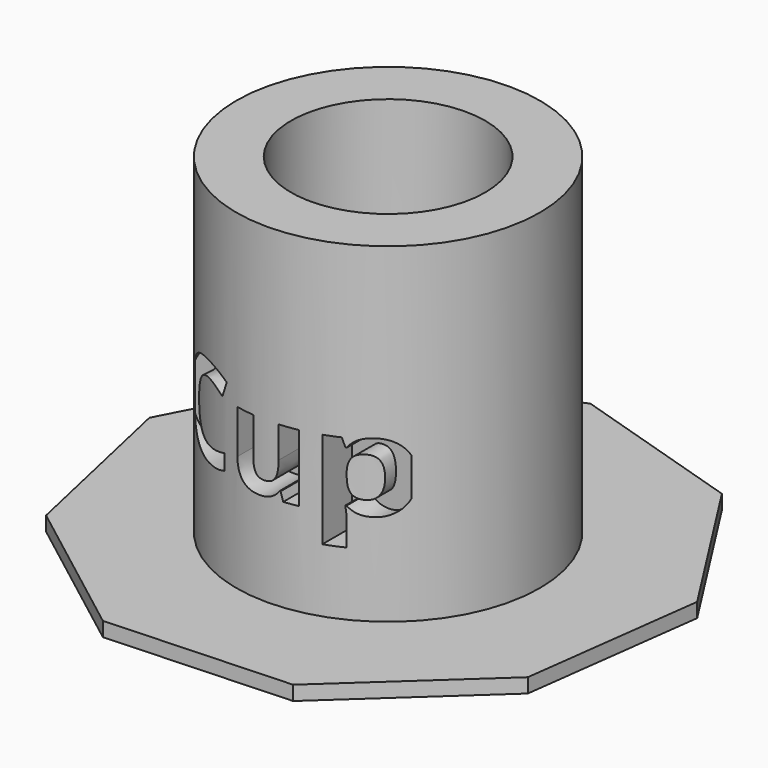
from build123d import *

# Parameters (mm, degrees)
F0_R         = 67.0452350449
F1_DEPTH     = 152.4
F2_T         = -24.13
F4_TEXT_SIZE = 54.2367187639
F5_DEPTH     = 21.59
F7_DEPTH     = 6.35


# Not quite as in the source:
# - a feature names something its author has since deleted; it is built from what else it names
# - Text() gives the source's letters only with a copy of the font that has no kerning and outlines rounded to 1/6400 em; it was checked with that copy


with BuildPart() as f1:
    # F0 (on Top) → F1 (new body)
    with BuildSketch(Plane.XY):
        Circle(F0_R)
    extrude(amount=F1_DEPTH)

    # F2
    f2_openings = [f1.faces().sort_by_distance(p)[0] for p in [
        (0, 0, 152.4),
    ]]
    offset(amount=F2_T, openings=f2_openings)

    # F4 (on offset) → F5 (cut)
    with BuildSketch(Plane.XZ.offset(68.58)):
        with Locations((-52.7822864242, 47.4721044302)):
            Text('Cup', F4_TEXT_SIZE, font='Open Sans', font_style=FontStyle.BOLD, text_align=(TextAlign.LEFT, TextAlign.BOTTOM))
    extrude(amount=-F5_DEPTH, mode=Mode.SUBTRACT)

    # F6 (on Top) → F7 (join)
    with BuildSketch(Plane.XY):
        Polygon((45.6455062393, -109.535330228), (105.3744395014, -54.5685651978), (115.7975014144, 25.9314379504), (72.0376254697, 94.2978330858), (-5.4294560413, 118.5412241167), (-80.3560347289, 87.3178589444), (-117.683131709, 15.2374971422), (-99.9449834601, -63.9726589188), (-35.4414666855, -113.2492968948), align=None)
    extrude(amount=F7_DEPTH)


solid = f1.part
